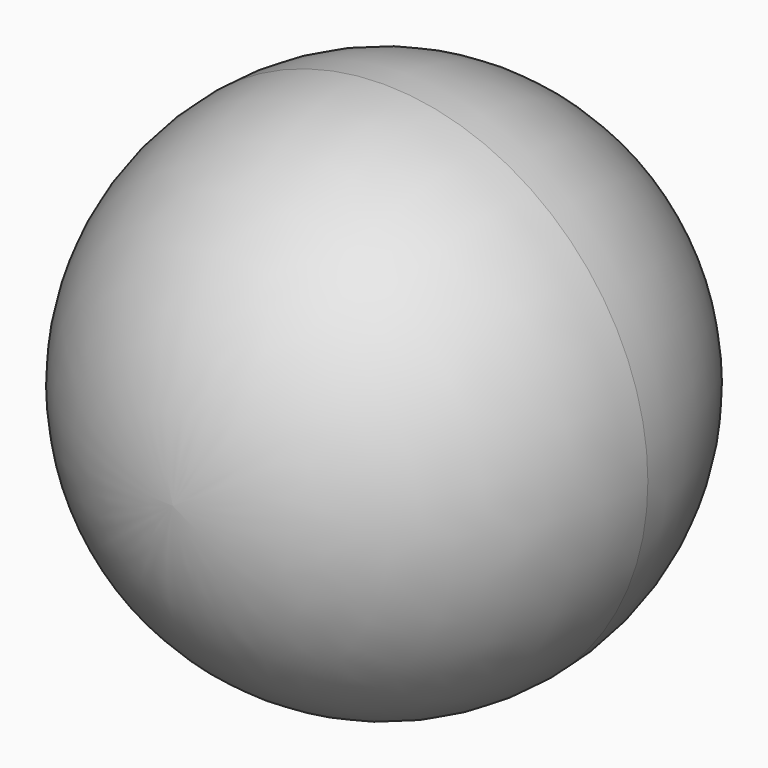
from build123d import *

# Parameters (mm, degrees)
F0_R     = 7.5
F1_DEPTH = 7.5
F2_R     = 7.49999
F3_DEPTH = 7.5
F4_R     = 7.49999


# Not quite as in the source:
# - a fillet or chamfer is up to 0.001 mm smaller than in the source, because OpenCascade refuses the exact size


with BuildPart() as f1:
    # F0 (on Front) → F1 (new body)
    with BuildSketch(Plane.XZ):
        Circle(F0_R)
    extrude(amount=F1_DEPTH)

    # F2 (radius 7.5 in the source; OpenCascade refuses exactly that, so slightly less here)
    f2_edges = [f1.edges().sort_by_distance(p)[0] for p in [
        (-7.5, -7.5, 0),
    ]]
    fillet(f2_edges, radius=F2_R)

    # F3 (add): a face of the model
    f3_faces = [f1.faces().sort_by_distance(p)[0] for p in [
        (0, 0, 0),
    ]]
    extrude(f3_faces, amount=F3_DEPTH)

    # F4 (radius 7.5 in the source; OpenCascade refuses exactly that, so slightly less here)
    f4_edges = [f1.edges().sort_by_distance(p)[0] for p in [
        (-7.5, 7.5, 0),
    ]]
    fillet(f4_edges, radius=F4_R)


solid = f1.part
